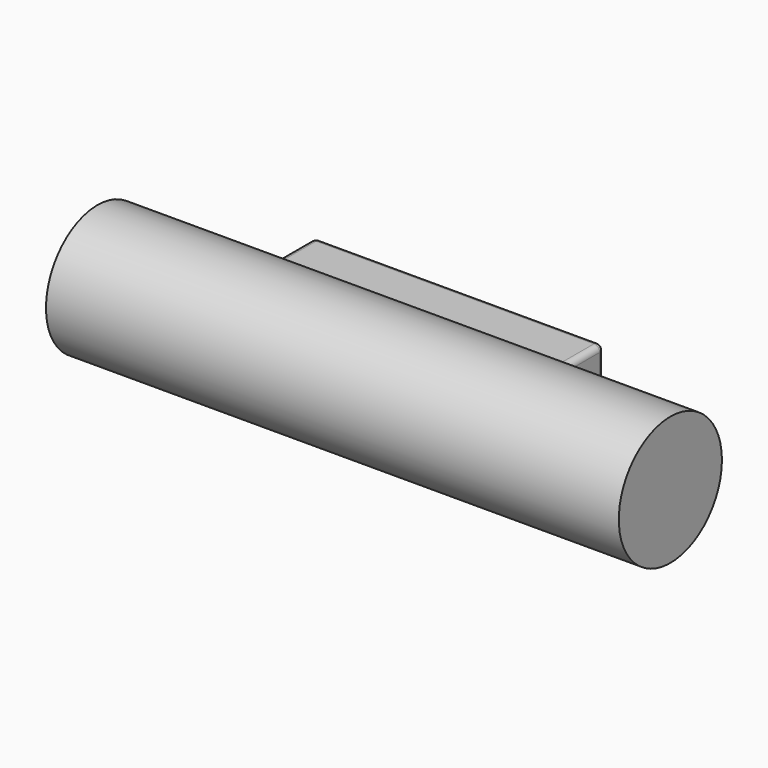
from build123d import *

# Parameters (mm, degrees)
F0_R     = 22.5
F1_DEPTH = 100
F2_DEPTH = 47.5
F3_W     = 101
F3_H     = 31
F3_W_2   = 95
F3_H_2   = 25
F4_DEPTH = 25
F5_R     = 2


with BuildPart() as f1:
    # F0 (on Right) → F1 (new body, symmetric)
    with BuildSketch(Plane.YZ):
        with Locations((-22.5, 0)):
            Circle(F0_R)
    extrude(amount=F1_DEPTH, both=True)


with BuildPart() as f2:
    # F0 (on Right) → F2 (new body, symmetric)
    with BuildSketch(Plane.YZ):
        Polygon((0, 12.5), (0, 0), (0, -12.5), (10.5, -12.5), (10.5, 12.5), align=None)
    extrude(amount=F2_DEPTH, both=True)


with BuildPart() as f4:
    # F3 (on face) → F4 (new body)
    with BuildSketch(Plane(origin=(0, 10.5, 0), x_dir=(-1, 0, 0), z_dir=(0, 1, 0))):
        Rectangle(F3_W, F3_H)
        Rectangle(F3_W_2, F3_H_2, mode=Mode.SUBTRACT)
    extrude(amount=-F4_DEPTH)

    # F5
    f5_edges = [f4.edges().sort_by_distance(p)[0] for p in [
        (50.5, -2, 15.5),
        (50.5, -2, -15.5),
        (-50.5, -2, 15.5),
        (-50.5, -2, -15.5),
        (0, 10.5, 15.5),
        (50.5, 10.5, 0),
        (0, 10.5, -15.5),
        (-50.5, 10.5, 0),
    ]]
    fillet(f5_edges, radius=F5_R)


solid = Compound([f1.part, f2.part, f4.part])
